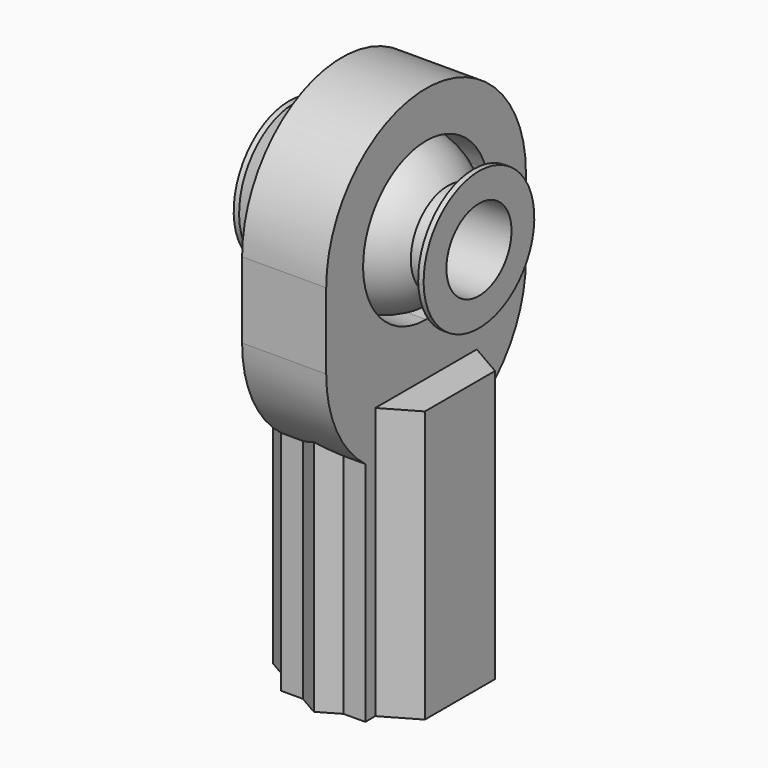
from build123d import *

# Parameters (mm, degrees)
F2_R     = 1.5
F3_DEPTH = 7.001
F5_DEPTH = 1.55
F7_DEPTH = 10
F6_R     = 1.25
F8_DEPTH = 7


# Not quite as in the source:
# - a feature names something its author has since deleted; it is built from what else it names


with BuildPart() as f1:
    # F0 (on Front) → F1 (revolve)
    with BuildSketch(Plane.XZ):
        with BuildLine():
            ThreePointArc((2.3494680249, 1.7), (2.7589361421, 0.8934603315), (2.9, 0))
            Line((2.9, 0), (3.5, 0))
            Line((3.5, 0), (3.5, 2.55))
            Line((3.5, 2.55), (3.3, 2.55))
            Line((3.3, 2.55), (2.9305491433, 1.7))
            Line((2.9305491433, 1.7), (2.3494680249, 1.7))
        make_face()
        with BuildLine():
            Line((-2.9, 0), (2.9, 0))
            ThreePointArc((2.9, 0), (2.7589361421, 0.8934603315), (2.3494680249, 1.7))
            ThreePointArc((2.3494680249, 1.7), (0, 2.9), (-2.3494680249, 1.7))
            ThreePointArc((-2.3494680249, 1.7), (-2.7589361421, 0.8934603315), (-2.9, 0))
        make_face()
        with BuildLine():
            Line((-3.5, 0), (-2.9, 0))
            ThreePointArc((-2.9, 0), (-2.7589361421, 0.8934603315), (-2.3494680249, 1.7))
            Line((-2.3494680249, 1.7), (-2.9305491433, 1.7))
            Line((-2.9305491433, 1.7), (-3.3, 2.55))
            Line((-3.3, 2.55), (-3.5, 2.55))
            Line((-3.5, 2.55), (-3.5, 0))
        make_face()
    revolve(axis=Axis((1.75, 0, 0), (1, 0, 0)))

    # F2 (on face) → F3 (cut, through all)
    with BuildSketch(Plane(origin=(-3.5, 0, 0), x_dir=(0, -1, 0), z_dir=(-1, 0, 0))):
        Circle(F2_R)
    extrude(amount=-F3_DEPTH, mode=Mode.SUBTRACT)


with BuildPart() as f5:
    # F4 (on Right) → F5 (new body, symmetric)
    with BuildSketch(Plane.YZ):
        with BuildLine():
            ThreePointArc((4.38178046, -1.4), (4.5451177166, -0.708452498), (4.6, 0))
            ThreePointArc((4.6, 0), (0, 4.6), (-4.6, 0))
            ThreePointArc((-4.6, 0), (-4.5451177166, -0.708452498), (-4.38178046, -1.4))
            ThreePointArc((-4.38178046, -1.4), (-3.7499980255, -0.1358838598), (-2.7642805233, 0.8767857143))
            ThreePointArc((-2.7642805233, 0.8767857143), (-1.7127932491, 2.3401579617), (0, 2.9))
            ThreePointArc((0, 2.9), (1.7127932491, 2.3401579617), (2.7642805233, 0.8767857143))
            ThreePointArc((2.7642805233, 0.8767857143), (3.7499980255, -0.1358838598), (4.38178046, -1.4))
        make_face()
        with BuildLine():
            ThreePointArc((-2.8, -3.6496575182), (-3.7629419848, -2.6458018858), (-4.38178046, -1.4))
            ThreePointArc((-4.38178046, -1.4), (-4.5451177166, -2.091547502), (-4.6, -2.8))
            ThreePointArc((-4.6, -2.8), (-4.1255302689, -4.8346989949), (-2.8, -6.4496575182))
            Line((-2.8, -6.4496575182), (-2.8, -3.6496575182))
        make_face()
        with BuildLine():
            ThreePointArc((-4.38178046, -1.4), (-4.5451177166, -0.708452498), (-4.6, 0))
            Line((-4.6, 0), (-4.6, -2.8))
            ThreePointArc((-4.6, -2.8), (-4.5451177166, -2.091547502), (-4.38178046, -1.4))
        make_face()
        with BuildLine():
            Line((4.6, -2.8), (4.6, 0))
            ThreePointArc((4.6, 0), (4.5451177166, -0.708452498), (4.38178046, -1.4))
            ThreePointArc((4.38178046, -1.4), (4.5451177166, -2.091547502), (4.6, -2.8))
        make_face()
        with BuildLine():
            ThreePointArc((-2.7642805233, 0.8767857143), (-3.7499980255, -0.1358838598), (-4.38178046, -1.4))
            ThreePointArc((-4.38178046, -1.4), (-3.7629419848, -2.6458018858), (-2.8, -3.6496575182))
            Line((-2.8, -3.6496575182), (-2.8, -0.7549834435))
            ThreePointArc((-2.8, -0.7549834435), (-2.8993054481, 0.0634658849), (-2.7642805233, 0.8767857143))
        make_face()
        with BuildLine():
            Line((2.8, -14.8188183084), (2.8, -6.4496575182))
            ThreePointArc((2.8, -6.4496575182), (0, -7.4), (-2.8, -6.4496575182))
            Line((-2.8, -6.4496575182), (-2.8, -14.8188183084))
            Line((-2.8, -14.8188183084), (0, -14.8188183084))
            Line((0, -14.8188183084), (2.8, -14.8188183084))
        make_face()
        with BuildLine():
            Line((2.8, -6.4496575182), (2.8, -3.6496575182))
            ThreePointArc((2.8, -3.6496575182), (0, -4.6), (-2.8, -3.6496575182))
            Line((-2.8, -3.6496575182), (-2.8, -6.4496575182))
            ThreePointArc((-2.8, -6.4496575182), (0, -7.4), (2.8, -6.4496575182))
        make_face()
        with BuildLine():
            ThreePointArc((-2.8, -3.6496575182), (0, -4.6), (2.8, -3.6496575182))
            Line((2.8, -3.6496575182), (2.8, -0.7549834435))
            ThreePointArc((2.8, -0.7549834435), (1.7635968947, -2.3021133754), (0, -2.9))
            ThreePointArc((0, -2.9), (-1.7635968947, -2.3021133754), (-2.8, -0.7549834435))
            Line((-2.8, -0.7549834435), (-2.8, -3.6496575182))
        make_face()
        with BuildLine():
            ThreePointArc((4.6, -2.8), (4.5451177166, -2.091547502), (4.38178046, -1.4))
            ThreePointArc((4.38178046, -1.4), (3.7629419848, -2.6458018858), (2.8, -3.6496575182))
            Line((2.8, -3.6496575182), (2.8, -6.4496575182))
            ThreePointArc((2.8, -6.4496575182), (4.1255302689, -4.8346989949), (4.6, -2.8))
        make_face()
        with BuildLine():
            ThreePointArc((2.8, -3.6496575182), (3.7629419848, -2.6458018858), (4.38178046, -1.4))
            ThreePointArc((4.38178046, -1.4), (3.7499980255, -0.1358838598), (2.7642805233, 0.8767857143))
            ThreePointArc((2.7642805233, 0.8767857143), (2.865869285, 0.4436138425), (2.9, 0))
            ThreePointArc((2.9, 0), (2.8748913023, -0.3807886553), (2.8, -0.7549834435))
            Line((2.8, -0.7549834435), (2.8, -3.6496575182))
        make_face()
    extrude(amount=F5_DEPTH, both=True)

    # F6 (on face) → F7 (join)
    with BuildSketch(Plane(origin=(0, 0, -14.8188183084), x_dir=(1, 0, 0), z_dir=(0, 0, -1))):
        Polygon((-2.8, 1.6165807537), (-2.8, -1.6165807537), (-1.55, -2.3382685902), (-1.55, 2.3382685902), align=None)
        Polygon((0, 3.2331615075), (-0.7502577388, 2.8), (0.7502577388, 2.8), align=None)
        Polygon((1.55, 2.3382685902), (1.55, -2.3382685902), (2.8, -1.6165807537), (2.8, 1.6165807537), align=None)
        Polygon((0.7502577388, -2.8), (-0.7502577388, -2.8), (0, -3.2331615075), align=None)
    extrude(amount=-F7_DEPTH)

    # F6 (on face) → F8 (cut)
    with BuildSketch(Plane(origin=(0, 0, -14.8188183084), x_dir=(1, 0, 0), z_dir=(0, 0, -1))):
        Circle(F6_R)
    extrude(amount=-F8_DEPTH, mode=Mode.SUBTRACT)


solid = Compound([f1.part, f5.part])
